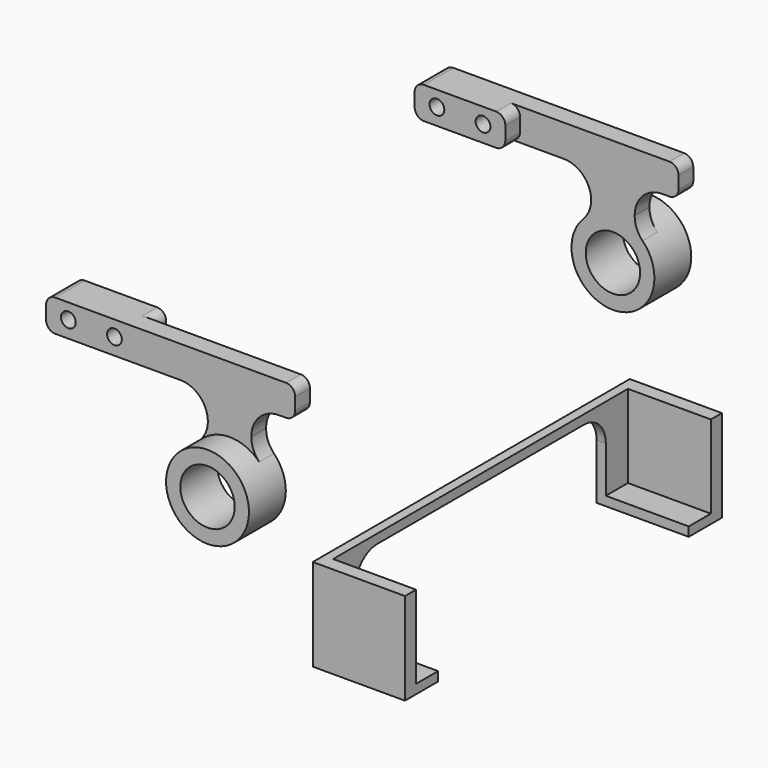
from build123d import *

# Parameters (mm, degrees)
F0_R        = 2.95
F0_R_2      = 0.8
F0_W        = 4.7585960214
F0_H        = 3.3378887317
F1_DEPTH    = 2
F2_W        = 9.8369888743
F2_H        = 3.4630449291
F2_R        = 0.8
F3_DEPTH    = 2
F4_DEPTH    = 5
F5_T1_DEPTH = 2
F6_R        = 1
F10_W       = 3
F10_H       = 8
F10_H_2     = 1
F11_DEPTH   = 1
F12_DEPTH   = 10
F13_R       = 3


# Not quite as in the source:
# - a fillet or chamfer that OpenCascade refuses, or shapes differently, is made with other operations: its cross-section is extruded or revolved along the edge and cut away or added


with BuildPart() as f1:
    # F0 (on Front) → F1 (new body)
    with BuildSketch(Plane.XZ):
        with BuildLine():
            ThreePointArc((-2.3600532936, 3.8314681848), (-2.1942835025, -3.9287555168), (4.5, 0))
            ThreePointArc((4.5, 0), (3.9287555168, 2.1942835025), (2.3600532936, 3.8314681848))
            ThreePointArc((2.3600532936, 3.8314681848), (0, 4.5), (-2.3600532936, 3.8314681848))
        make_face()
        Circle(F0_R, mode=Mode.SUBTRACT)
        with BuildLine():
            ThreePointArc((-2.3600532936, 3.8314681848), (0, 4.5), (2.3600532936, 3.8314681848))
            Line((2.3600532936, 3.8314681848), (2.3600532936, 6.6316658631))
            Line((2.3600532936, 6.6316658631), (-2.3600532936, 6.6316658631))
            Line((-2.3600532936, 6.6316658631), (-2.3600532936, 3.8314681848))
        make_face()
        Polygon((-2.3600532936, 6.6316658631), (2.3600532936, 6.6316658631), (2.3600532936, 8.3240726963), (2.3600532936, 11.6619614279), (-19.9184944371, 11.6619614279), (-19.9184944371, 8.1989164988), (-2.3600532936, 8.1989164988), align=None)
        with Locations((-17.5, 10)):
            Circle(F0_R_2, mode=Mode.SUBTRACT)
        with Locations((-12.5, 10)):
            Circle(F0_R_2, mode=Mode.SUBTRACT)
        with Locations((4.7393513044, 9.9930170621)):
            Rectangle(F0_W, F0_H)
    extrude(amount=F1_DEPTH)

    # F2 (on face) → F3 (join)
    with BuildSketch(Plane(origin=(0, 0, 0), x_dir=(-1, 0, 0), z_dir=(0, 1, 0))):
        with Locations((15, 9.9304389634)):
            Rectangle(F2_W, F2_H)
        with Locations((12.5, 10)):
            Circle(F2_R, mode=Mode.SUBTRACT)
        with Locations((17.5, 10)):
            Circle(F2_R, mode=Mode.SUBTRACT)
    extrude(amount=F3_DEPTH)

    # F0 (on Front) → F4 (join)
    with BuildSketch(Plane.XZ):
        with BuildLine():
            ThreePointArc((-2.3600532936, 3.8314681848), (-2.1942835025, -3.9287555168), (4.5, 0))
            ThreePointArc((4.5, 0), (3.9287555168, 2.1942835025), (2.3600532936, 3.8314681848))
            ThreePointArc((2.3600532936, 3.8314681848), (0, 4.5), (-2.3600532936, 3.8314681848))
        make_face()
        Circle(F0_R, mode=Mode.SUBTRACT)
    extrude(amount=F4_DEPTH)

    # F5: fillet of radius 3 on 4 edges, made by hand

    # F5_s2 → F5_t1 (join)
    with BuildSketch(Plane.XZ):
        with BuildLine():
            ThreePointArc((3.2160319762, 3.1475606949), (2.582278649, 4.1128113633), (2.3600532936, 5.2459344915))
            Line((2.3600532936, 5.2459344915), (2.3600532936, 3.8314681848))
            ThreePointArc((2.3600532936, 3.8314681848), (2.8089346909, 3.5156629392), (3.2160319762, 3.1475606949))
        make_face()
        with BuildLine():
            ThreePointArc((-5.3600532936, 8.1989164988), (-3.2387329501, 7.3202368424), (-2.3600532936, 5.1989164988))
            Line((-2.3600532936, 5.1989164988), (-2.3600532936, 8.1989164988))
            Line((-2.3600532936, 8.1989164988), (-5.3600532936, 8.1989164988))
        make_face()
        with BuildLine():
            ThreePointArc((-3.2160319762, 3.1475606949), (-2.582278649, 4.1128113633), (-2.3600532936, 5.2459344915))
            Line((-2.3600532936, 5.2459344915), (-2.3600532936, 3.8314681848))
            ThreePointArc((-2.3600532936, 3.8314681848), (-2.8089346909, 3.5156629392), (-3.2160319762, 3.1475606949))
        make_face()
        with BuildLine():
            ThreePointArc((2.3600532936, 5.3240726963), (3.2387329501, 7.4453930398), (5.3600532936, 8.3240726963))
            Line((5.3600532936, 8.3240726963), (2.3600532936, 8.3240726963))
            Line((2.3600532936, 8.3240726963), (2.3600532936, 5.3240726963))
        make_face()
    extrude(amount=F5_T1_DEPTH)

    # F6
    f6_edges = [f1.edges().sort_by_distance(p)[0] for p in [
        (-19.918494, 0, 11.661961),
        (-10.081506, 1, 11.661961),
        (-19.918494, 0, 8.198916),
        (-10.081506, 1, 8.198916),
        (7.118649, -1, 8.324073),
        (7.118649, -1, 11.661961),
    ]]
    fillet(f6_edges, radius=F6_R)


with BuildPart() as f8_1:
    # F8: instance of F1
    add(f1.part.mirror(Plane.XZ.offset(-25)))


with BuildPart() as f11:
    # F10 (on offset) → F11 (new body)
    with BuildSketch(Plane.YZ.offset(25)):
        Polygon((-20.4657563084, 8.8006782488), (-21.9657563084, 8.8006782488), (-21.9657563084, -1.1993217512), (-20.4657563084, -1.1993217512), (-20.4657563084, -0.1993217512), (-20.4657563084, 7.8006782488), align=None)
        Polygon((19.5342436916, 8.8006782488), (-20.4657563084, 8.8006782488), (-20.4657563084, 7.8006782488), (-17.4657563084, 7.8006782488), (16.5342436916, 7.8006782488), (19.5342436916, 7.8006782488), align=None)
        with Locations((-18.9657563084, 3.8006782488)):
            Rectangle(F10_W, F10_H)
        Polygon((21.0342436916, 8.8006782488), (19.5342436916, 8.8006782488), (19.5342436916, 7.8006782488), (19.5342436916, -0.1993217512), (19.5342436916, -1.1993217512), (21.0342436916, -1.1993217512), align=None)
        with Locations((-18.9657563084, -0.6993217512)):
            Rectangle(F10_W, F10_H_2)
        with Locations((18.0342436916, 3.8006782488)):
            Rectangle(F10_W, F10_H)
        with Locations((18.0342436916, -0.6993217512)):
            Rectangle(F10_W, F10_H_2)
    extrude(amount=F11_DEPTH)

    # F10 (on offset) → F12 (join)
    with BuildSketch(Plane.YZ.offset(25)):
        with Locations((18.0342436916, -0.6993217512)):
            Rectangle(F10_W, F10_H_2)
        with Locations((-18.9657563084, -0.6993217512)):
            Rectangle(F10_W, F10_H_2)
        Polygon((21.0342436916, 8.8006782488), (19.5342436916, 8.8006782488), (19.5342436916, 7.8006782488), (19.5342436916, -0.1993217512), (19.5342436916, -1.1993217512), (21.0342436916, -1.1993217512), align=None)
        Polygon((-20.4657563084, 8.8006782488), (-21.9657563084, 8.8006782488), (-21.9657563084, -1.1993217512), (-20.4657563084, -1.1993217512), (-20.4657563084, -0.1993217512), (-20.4657563084, 7.8006782488), align=None)
    extrude(amount=F12_DEPTH)

    # F13
    f13_edges = [f11.edges().sort_by_distance(p)[0] for p in [
        (25.5, 16.534244, 7.800678),
        (25.5, -17.465756, 7.800678),
    ]]
    fillet(f13_edges, radius=F13_R)


solid = Compound([f1.part, f8_1.part, f11.part])
